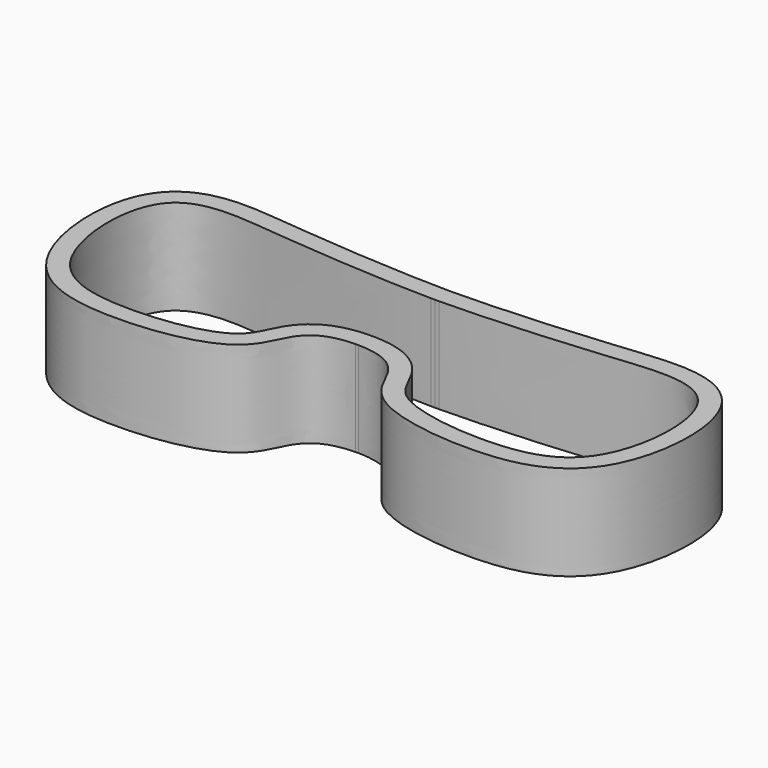
from build123d import *

# Parameters (mm, degrees)
F1_DEPTH = 25.4


# Not quite as in the source:
# - the dataset's text gives a spline's control points without its knots; the knots are read off the source's solid


with BuildPart() as f1:
    # F0 (on Top) → F1 (new body)
    with BuildSketch(Plane.XY):
        with BuildLine():
            add(Edge.make_bspline(
                [(0, 37.9999992061), (-0.3553457346, 37.9999992468), (-0.7175293681, 38.0011693983), (-1.0860350785, 38.0034641742)],
                knots=[0, 0, 0, 0, 0.0067263179, 0.0067263179, 0.0067263179, 0.0067263179], degree=3))
            add(Edge.make_bspline(
                [(0, 37.9999992061), (0.3553454825, 37.9999992468), (0.7175288542, 38.0011693966), (1.0860342942, 38.0034641693)],
                knots=[0, 0, 0, 0, 0.0067263132, 0.0067263132, 0.0067263132, 0.0067263132], degree=3))
            add(Edge.make_bspline(
                [(1.0860342943, 38.0034641693), (0.9347367621, 40.0800248778), (0.7277247884, 41.822412903), (0.4623789025, 43.0006673854)],
                knots=[0.98882329, 0.98882329, 0.98882329, 0.98882329, 0.996172688, 0.996172688, 0.996172688, 0.996172688], degree=3))
            add(Edge.make_bspline(
                [(-4.833e-07, 42.9999992067), (0.1526808368, 42.9999992247), (0.3068243562, 43.0002231121), (0.4623789021, 43.0006673852)],
                knots=[3.7e-09, 3.7e-09, 3.7e-09, 3.7e-09, 0.0029822166, 0.0029822166, 0.0029822166, 0.0029822166], degree=3))
            add(Edge.make_bspline(
                [(-4.841e-07, 42.9999992067), (-0.1526817916, 42.9999992247), (-0.3068252979, 43.0002231121), (-0.4623798303, 43.0006673851)],
                knots=[3.7e-09, 3.7e-09, 3.7e-09, 3.7e-09, 0.0029822163, 0.0029822163, 0.0029822163, 0.0029822163], degree=3))
            add(Edge.make_bspline(
                [(-1.0860350786, 38.0034641742), (-0.9347376061, 40.0800248804), (-0.7277256825, 41.8224129037), (-0.4623798308, 43.0006673853)],
                knots=[0.98882329, 0.98882329, 0.98882329, 0.98882329, 0.996172688, 0.996172688, 0.996172688, 0.996172688], degree=3))
        make_face()
        with BuildLine():
            add(Edge.make_bspline(
                [(-1.0860350785, 38.0034641742), (-7.9140986977, 38.0459842091), (-26.1218890397, 38.9132812222), (-46.6825788281, 40.8149720811), (-77.5540911423, 44.0015899948), (-75.3755129326, 0.3195886834), (-51.0502450403, -7.0483658316), (-21.0290096408, -2.6626653392), (-18.3123324837, 9.1336067711), (-10.8329689555, 16.693589117), (-1.0510685803, 16.9845771948)],
                knots=[0.0067263179, 0.0067263179, 0.0067263179, 0.0067263179, 0.1313586521, 0.2589077893, 0.3863117478, 0.5348226679, 0.6623089336, 0.8004731597, 0.8832955389, 0.9960402045, 0.9960402045, 0.9960402045, 0.9960402045], degree=3))
            add(Edge.make_bspline(
                [(-1.0860350786, 38.0034641742), (-0.9347376061, 40.0800248804), (-0.7277256825, 41.8224129037), (-0.4623798308, 43.0006673853)],
                knots=[0.98882329, 0.98882329, 0.98882329, 0.98882329, 0.996172688, 0.996172688, 0.996172688, 0.996172688], degree=3))
            add(Edge.make_bspline(
                [(-0.4623798303, 43.0006673851), (-1.9368494382, 43.0048785582), (-5.3082727542, 43.055436398), (-11.0123417341, 43.2463517355), (-16.1576550023, 43.4911770463), (-20.2544329187, 43.7216088449), (-23.2793616831, 43.9083770562), (-26.2093976008, 44.105136), (-29.9932125292, 44.3798009503), (-33.6624712277, 44.6756225434), (-37.3322790813, 44.9964761321), (-40.1145812272, 45.2506871777), (-42.9550981039, 45.5193616659), (-45.396461039, 45.7563883607), (-47.4042849577, 45.9537346264), (-49.4671103205, 46.1584839724), (-52.1841644839, 46.4117809706), (-55.5802616826, 46.6253874644), (-59.0634610919, 46.658181629), (-62.5915601724, 46.4049484922), (-66.1295051147, 45.7349627405), (-69.0415772799, 44.6844641947), (-71.2771347205, 43.4509073335), (-72.8742907086, 42.3100315751), (-74.1056828131, 41.1746403412), (-75.0152359089, 40.1537375097), (-75.8553242208, 39.0775722969), (-76.7692402802, 37.6580237594), (-77.9786551326, 35.2590509425), (-79.0734299323, 32.0706122875), (-79.8537449717, 28.0286085075), (-80.1749064509, 23.8407820813), (-80.0803146303, 19.5836272999), (-79.5952719389, 15.3395269981), (-78.7325024229, 11.1937779604), (-77.6989835122, 7.8913141079), (-76.6726143501, 5.3810666312), (-75.7976977702, 3.5744085116), (-74.8064622775, 1.8530478679), (-73.7117847903, 0.2541474713), (-72.5163439774, -1.2231947396), (-70.7968330684, -3.0244512037), (-68.4328545365, -4.9526596116), (-65.3392499159, -6.7520959101), (-62.0706703277, -8.0819207464), (-58.6811747661, -9.0110168251), (-55.1993808792, -9.6122497915), (-52.229803237, -9.8951878123), (-49.8198692869, -10.0195683838), (-47.3737039644, -10.0839106844), (-44.2611046598, -10.052799743), (-40.5009296651, -9.8406289829), (-36.7775972695, -9.4542038323), (-33.152231348, -8.8913371785), (-29.6819932106, -8.1454776655), (-26.4166328268, -7.2011932762), (-23.8976820718, -6.2228230842), (-22.0137606932, -5.2863060297), (-20.6694427133, -4.4914039285), (-19.3924216601, -3.5694580552), (-18.2711084165, -2.571223159), (-17.3010092404, -1.5213343193), (-16.4812288846, -0.4544223389), (-15.7962398553, 0.5965147313), (-15.0322527333, 1.94239018), (-14.2897907816, 3.4749732704), (-13.6687742713, 4.7732335166), (-13.1794454653, 5.6865594363), (-12.7939767922, 6.3338225494), (-12.3733495353, 6.9619883036), (-11.7646404109, 7.7627118612), (-10.9005577404, 8.69374016), (-9.639520854, 9.6977253648), (-8.0546712534, 10.5879104378), (-6.0184345269, 11.3328207927), (-3.5148922414, 11.8380466557), (-1.4877810143, 11.9817980997), (-0.4476397786, 11.9967968232)],
                knots=[0.0029822163, 0.0029822163, 0.0029822163, 0.0029822163, 0.03125, 0.0625, 0.09375, 0.109375, 0.125, 0.140625, 0.15625, 0.1875, 0.203125, 0.21875, 0.234375, 0.25, 0.2578125, 0.265625, 0.28125, 0.296875, 0.3125, 0.328125, 0.34375, 0.359375, 0.3671875, 0.375, 0.3828125, 0.38671875, 0.390625, 0.3984375, 0.40625, 0.421875, 0.4375, 0.453125, 0.46875, 0.484375, 0.5, 0.515625, 0.5234375, 0.53125, 0.5390625, 0.546875, 0.5546875, 0.5625, 0.578125, 0.59375, 0.609375, 0.625, 0.640625, 0.65625, 0.6640625, 0.671875, 0.6875, 0.703125, 0.71875, 0.734375, 0.75, 0.765625, 0.78125, 0.7890625, 0.796875, 0.8046875, 0.8125, 0.8203125, 0.828125, 0.8359375, 0.84375, 0.859375, 0.875, 0.8828125, 0.890625, 0.8984375, 0.90625, 0.921875, 0.9375, 0.953125, 0.96875, 0.984375, 0.9980614265, 0.9980614265, 0.9980614265, 0.9980614265], degree=3))
            add(Edge.make_bspline(
                [(-0.4476397944, 11.9967968167), (-0.6958884993, 13.1586870358), (-0.8979274286, 14.8999393719), (-1.05106858, 16.9845771948)],
                knots=[0.9599433574, 0.9599433574, 0.9599433574, 0.9599433574, 0.9673562913, 0.9673562913, 0.9673562913, 0.9673562913], degree=3))
        make_face()
        with BuildLine():
            add(Edge.make_bspline(
                [(1.0860342943, 38.0034641693), (0.9347367621, 40.0800248778), (0.7277247884, 41.822412903), (0.4623789025, 43.0006673854)],
                knots=[0.98882329, 0.98882329, 0.98882329, 0.98882329, 0.996172688, 0.996172688, 0.996172688, 0.996172688], degree=3))
            add(Edge.make_bspline(
                [(1.0860342942, 38.0034641693), (7.9140980086, 38.0459841763), (26.1218887812, 38.9132811983), (46.6825788281, 40.8149720811), (77.5540911423, 44.0015899948), (75.3755129326, 0.3195886834), (51.0502450403, -7.0483658316), (21.0290096408, -2.6626653392), (18.3123324781, 9.1336067958), (10.8329689022, 16.6935891708), (1.051068399, 16.9845772002)],
                knots=[0.0067263132, 0.0067263132, 0.0067263132, 0.0067263132, 0.1313586521, 0.2589077893, 0.3863117478, 0.5348226679, 0.6623089336, 0.8004731597, 0.8832955389, 0.9960402052, 0.9960402052, 0.9960402052, 0.9960402052], degree=3))
            add(Edge.make_bspline(
                [(0.4476397559, 11.9967968172), (0.6958884276, 13.1586870374), (0.8979273071, 14.8999393753), (1.0510683987, 16.9845772003)],
                knots=[0.9599433573, 0.9599433573, 0.9599433573, 0.9599433573, 0.9673562912, 0.9673562912, 0.9673562912, 0.9673562912], degree=3))
            add(Edge.make_bspline(
                [(0.4623789021, 43.0006673852), (1.9368485051, 43.0048785584), (5.3082718546, 43.0554363961), (11.012340959, 43.2463517256), (16.1576543754, 43.4911770288), (20.2544324055, 43.721608822), (23.2793612475, 43.9083770298), (26.209397229, 44.1051359713), (29.9932122107, 44.3798009189), (33.662470926, 44.6756225102), (37.3322787726, 44.9964760977), (40.1145809046, 45.2506871425), (42.9550977627, 45.5193616301), (45.3964606793, 45.7563883243), (47.4042845868, 45.9537345896), (49.4671099284, 46.1584839348), (52.1841640772, 46.411780939), (55.5802612687, 46.6253874491), (59.0634606796, 46.6581816401), (62.5915597675, 46.4049485412), (66.1295047225, 45.7349628418), (69.0415769058, 44.6844643553), (71.2771343718, 43.4509075495), (72.8742903861, 42.3100318347), (74.1056825196, 41.1746406353), (75.0152356408, 40.1537378315), (75.8553239883, 39.0775726312), (76.7692400841, 37.6580241085), (77.9786549889, 35.2590513062), (79.0734298398, 32.0706126622), (79.8537449278, 28.0286088876), (80.1749064471, 23.8407824597), (80.0803146608, 19.5836276694), (79.5952719997, 15.3395273516), (78.7325025112, 11.1937782915), (77.6989836225, 7.8913144157), (76.6726144784, 5.3810669178), (75.7976979129, 3.5744087819), (74.8064624345, 1.8530481177), (73.7117849594, 0.2541476988), (72.5163441577, -1.2231945338), (70.7968332617, -3.0244510269), (68.4328547415, -4.9526594703), (65.3392501276, -6.7520958071), (62.0706705405, -8.0819206752), (58.681174977, -9.0110167791), (55.1993810864, -9.6122497646), (52.2298034403, -9.8951877973), (49.819869487, -10.0195683761), (47.3737041623, -10.0839106834), (44.2611048518, -10.0527997495), (40.500929847, -9.8406289976), (36.7775974384, -9.4542038543), (33.1522315017, -8.8913372071), (29.6819933476, -8.1454777001), (26.4166329463, -7.2011933167), (23.8976821771, -6.2228231302), (22.0137607873, -5.2863060809), (20.6694428, -4.4914039851), (19.3924217362, -3.5694581163), (18.2711084799, -2.571223221), (17.3010092928, -1.5213343805), (16.4812289272, -0.4544223972), (15.79623989, 0.5965146771), (15.0322527599, 1.9423901322), (14.2897908024, 3.4749732307), (13.6687742896, 4.7732334829), (13.1794454822, 5.6865594066), (12.793976809, 6.3338225209), (12.373349551, 6.9619882775), (11.7646404246, 7.7627118388), (10.9005577505, 8.6937401429), (9.6395208589, 9.6977253538), (8.0546712539, 10.5879104316), (6.0184345249, 11.3328207899), (3.5148922299, 11.8380466569), (1.48778099, 11.9817981013), (0.4476397401, 11.9967968238)],
                knots=[0.0029822166, 0.0029822166, 0.0029822166, 0.0029822166, 0.03125, 0.0625, 0.09375, 0.109375, 0.125, 0.140625, 0.15625, 0.1875, 0.203125, 0.21875, 0.234375, 0.25, 0.2578125, 0.265625, 0.28125, 0.296875, 0.3125, 0.328125, 0.34375, 0.359375, 0.3671875, 0.375, 0.3828125, 0.38671875, 0.390625, 0.3984375, 0.40625, 0.421875, 0.4375, 0.453125, 0.46875, 0.484375, 0.5, 0.515625, 0.5234375, 0.53125, 0.5390625, 0.546875, 0.5546875, 0.5625, 0.578125, 0.59375, 0.609375, 0.625, 0.640625, 0.65625, 0.6640625, 0.671875, 0.6875, 0.703125, 0.71875, 0.734375, 0.75, 0.765625, 0.78125, 0.7890625, 0.796875, 0.8046875, 0.8125, 0.8203125, 0.828125, 0.8359375, 0.84375, 0.859375, 0.875, 0.8828125, 0.890625, 0.8984375, 0.90625, 0.921875, 0.9375, 0.953125, 0.96875, 0.984375, 0.9980614267, 0.9980614267, 0.9980614267, 0.9980614267], degree=3))
        make_face()
        with BuildLine():
            add(Edge.make_bspline(
                [(-1.0510685803, 16.9845771948), (-0.7075106384, 16.9947972197), (-0.3572051825, 17), (0, 17)],
                knots=[0.9960402045, 0.9960402045, 0.9960402045, 0.9960402045, 1, 1, 1, 1], degree=3))
            add(Edge.make_bspline(
                [(-0.4476397944, 11.9967968167), (-0.6958884993, 13.1586870358), (-0.8979274286, 14.8999393719), (-1.05106858, 16.9845771948)],
                knots=[0.9599433574, 0.9599433574, 0.9599433574, 0.9599433574, 0.9673562913, 0.9673562913, 0.9673562913, 0.9673562913], degree=3))
            add(Edge.make_bspline(
                [(-0.4476397786, 11.9967968232), (-0.3003120457, 11.9989212731), (-0.1511060789, 12), (0, 12)],
                knots=[0.9980614265, 0.9980614265, 0.9980614265, 0.9980614265, 1, 1, 1, 1], degree=3))
            add(Edge.make_bspline(
                [(0.4476397401, 11.9967968238), (0.3003120197, 11.9989212733), (0.1511060658, 12), (0, 12)],
                knots=[0.9980614267, 0.9980614267, 0.9980614267, 0.9980614267, 1, 1, 1, 1], degree=3))
            add(Edge.make_bspline(
                [(0.4476397559, 11.9967968172), (0.6958884276, 13.1586870374), (0.8979273071, 14.8999393753), (1.0510683987, 16.9845772003)],
                knots=[0.9599433573, 0.9599433573, 0.9599433573, 0.9599433573, 0.9673562912, 0.9673562912, 0.9673562912, 0.9673562912], degree=3))
            add(Edge.make_bspline(
                [(1.051068399, 16.9845772002), (0.7075105152, 16.9947972215), (0.3572051197, 17), (0, 17)],
                knots=[0.9960402052, 0.9960402052, 0.9960402052, 0.9960402052, 1, 1, 1, 1], degree=3))
        make_face()
    extrude(amount=F1_DEPTH)


solid = f1.part
